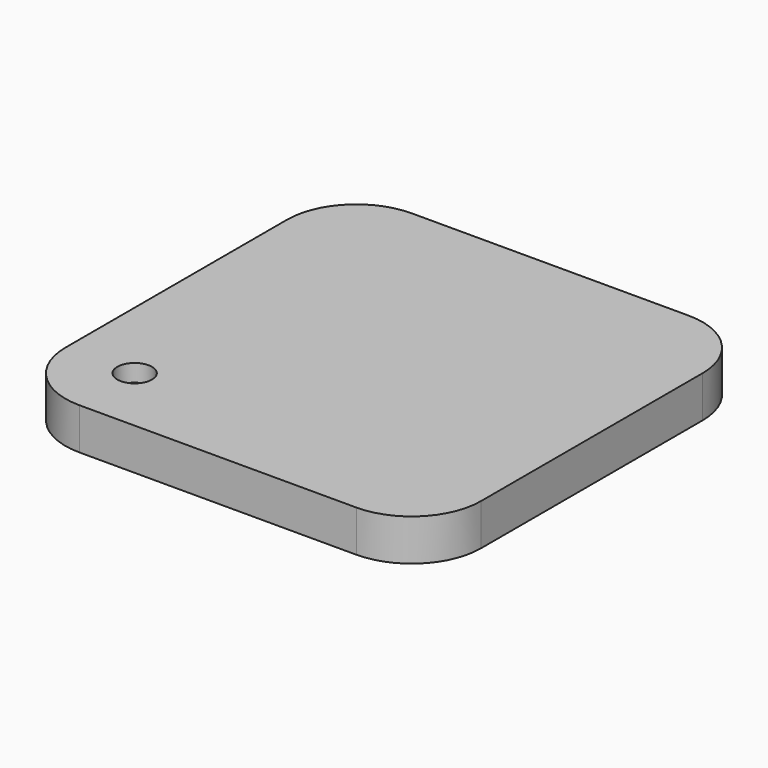
from build123d import *

# Parameters (mm, degrees)
F0_W         = 60
F0_H         = 60
F1_DEPTH     = 6
F2_R         = 10
F3_T         = -2.5
F4_TEXT_SIZE = 43.9755165846
F5_DEPTH     = 3
F7_D         = 5


# Not quite as in the source:
# - Text() gives the source's letters only with a copy of the font that has no kerning and outlines rounded to 1/6400 em; it was checked with that copy


with BuildPart() as f1:
    # F0 (on Top) → F1 (new body)
    with BuildSketch(Plane.XY):
        with Locations((5.494187586, -1.5848374665)):
            Rectangle(F0_W, F0_H)
    extrude(amount=F1_DEPTH)

    # F2
    f2_edges = [f1.edges().sort_by_distance(p)[0] for p in [
        (-24.505812, 28.415163, 3),
        (-24.505812, -31.584837, 3),
        (35.494188, -31.584837, 3),
        (35.494188, 28.415163, 3),
    ]]
    fillet(f2_edges, radius=F2_R)

    # F3
    f3_openings = [f1.faces().sort_by_distance(p)[0] for p in [
        (5.494188, -1.584837, 0),
    ]]
    offset(amount=F3_T, openings=f3_openings)

    # F4 (on face) → F5 (join)
    with BuildSketch(Plane(origin=(0, 0, 3.5), x_dir=(1, 0, 0), z_dir=(0, 0, -1))):
        with Locations((-21.9201052096, -14.8163661361)):
            Text('CT', F4_TEXT_SIZE, font='Open Sans', text_align=(TextAlign.LEFT, TextAlign.BOTTOM))
    extrude(amount=F5_DEPTH)

    # F7 (through all)
    with Locations(Plane(origin=(0, 0, 3.5), x_dir=(1, 0, 0), z_dir=(0, 0, -1))):
        with Locations((-14.505812414, 21.5848374665)):
            Hole(F7_D / 2)


solid = f1.part
